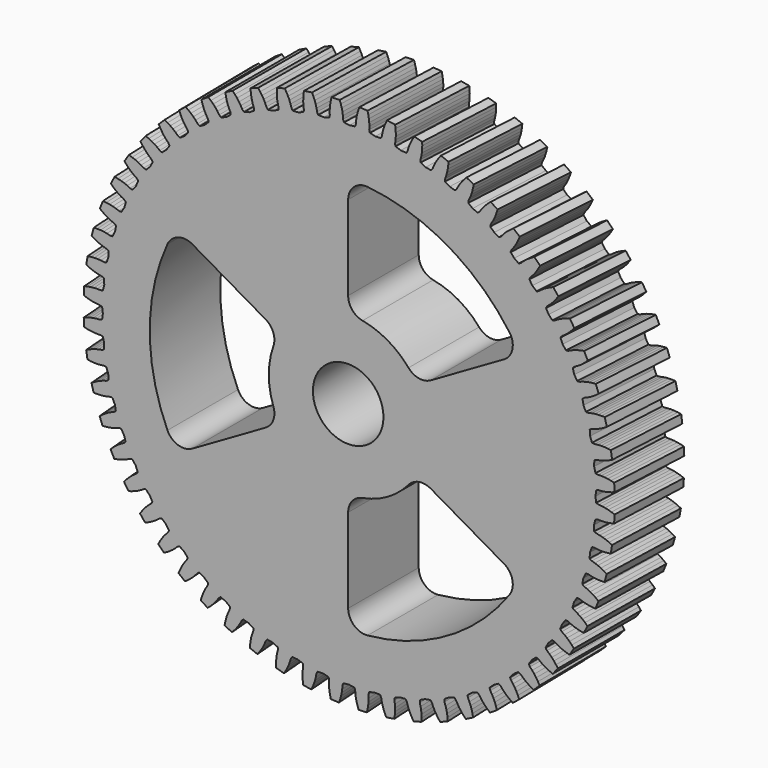
from build123d import *

# Parameters (mm, degrees)
F4_R     = 4
F5_DEPTH = 25
F7_DEPTH = 25


with BuildPart() as f3:
    # F0 (on Front) → F3 section 0
    with BuildSketch(Plane.XZ):
        Polygon((27.99593, -1.14699), (27.92323, -0.5264), (28.01927, 0.091), (28.1103, 0.13907), (28.29245, 0.18964), (28.65722, 0.21039), (29.02178, 0.25349), (29.38595, 0.32911), (29.74963, 0.42693), (30.11269, 0.54333), (30.08147, 1.47455), (29.71143, 1.56637), (29.34201, 1.63962), (28.9736, 1.69069), (28.60697, 1.70927), (28.24164, 1.70554), (28.0565, 1.74381), (27.96246, 1.78567), (27.82529, 2.39525), (27.85626, 3.01931), (27.94177, 3.07663), (28.11764, 3.14597), (28.47824, 3.20473), (28.8363, 3.2857), (29.19057, 3.39897), (29.54203, 3.53428), (29.89093, 3.68799), (29.76255, 4.61084), (29.38494, 4.66348), (29.00989, 4.69772), (28.63816, 4.70999), (28.27159, 4.69015), (27.90865, 4.64826), (27.72053, 4.66696), (27.62262, 4.69876), (27.42248, 5.29067), (27.38806, 5.91455), (27.4671, 5.98049), (27.63477, 6.06783), (27.98725, 6.16396), (28.33488, 6.28191), (28.67537, 6.4316), (29.01076, 6.6029), (29.34169, 6.79224), (29.11754, 7.69661), (28.7365, 7.7095), (28.35992, 7.70434), (27.98895, 7.67769), (27.62646, 7.61964), (27.26989, 7.54004), (27.08084, 7.53897), (26.98015, 7.56037), (26.71924, 8.12811), (26.61979, 8.74498), (26.69151, 8.81882), (26.84912, 8.92321), (27.18962, 9.05566), (27.52302, 9.2093), (27.846, 9.39376), (28.16165, 9.59918), (28.47097, 9.82207), (28.15352, 10.69806), (27.77321, 10.67105), (27.39924, 10.62655), (27.03308, 10.56127), (26.67865, 10.46565), (26.33235, 10.34922), (26.14445, 10.32839), (26.04208, 10.33914), (25.72325, 10.87651), (25.55986, 11.4796), (25.62347, 11.56053), (25.76931, 11.68082), (26.0941, 11.84814), (26.40962, 12.03579), (26.71154, 12.253), (27.00399, 12.49028), (27.28832, 12.74429), (26.88104, 13.5823), (26.50564, 13.51568), (26.13837, 13.43234), (25.78104, 13.32914), (25.43855, 13.197), (25.10631, 13.045), (24.92162, 13.00465), (24.81868, 13.00464), (24.44543, 13.50574), (24.2199, 14.08844), (24.2747, 14.17558), (24.40716, 14.31046), (24.71268, 14.51081), (25.00686, 14.73042), (25.28442, 14.97799), (25.55047, 15.24455), (25.80669, 15.52689), (25.31404, 16.31773), (24.94767, 16.21223), (24.59112, 16.09096), (24.24653, 15.95098), (23.91973, 15.78376), (23.6052, 15.59786), (23.42574, 15.53843), (23.32336, 15.52766), (22.89978, 15.98699), (22.61457, 16.54293), (22.65997, 16.63532), (22.77761, 16.78331), (23.06051, 17.0145), (23.33012, 17.26365), (23.58029, 17.53888), (23.81701, 17.83179), (24.04231, 18.13936), (23.4697, 18.87438), (23.11636, 18.73116), (22.77444, 18.57329), (22.44638, 18.39805), (22.13884, 18.19758), (21.84547, 17.97983), (21.6732, 17.90197), (21.57251, 17.88055), (21.10323, 18.29309), (20.76148, 18.81618), (20.79697, 18.9128), (20.8985, 19.07228), (21.15568, 19.33177), (21.39777, 19.60774), (21.6178, 19.90761), (21.82261, 20.22366), (22.01453, 20.5531), (21.36823, 21.22423), (21.03179, 21.04487), (20.70824, 20.85212), (20.40029, 20.64355), (20.1154, 20.41203), (19.84639, 20.16481), (19.68321, 20.06936), (19.58531, 20.03754), (19.07548, 20.39877), (18.68092, 20.88326), (18.70611, 20.98307), (18.79042, 21.15228), (19.01907, 21.43724), (19.23099, 21.737), (19.41846, 22.05823), (19.58911, 22.39395), (19.74555, 22.74165), (19.03263, 23.34155), (18.71678, 23.128), (18.41516, 22.90249), (18.1307, 22.66287), (17.87156, 22.40285), (17.62988, 22.12886), (17.47756, 22.01688), (17.38353, 21.975), (16.83873, 22.28095), (16.39569, 22.72155), (16.41031, 22.82345), (16.47647, 23.00054), (16.67408, 23.30784), (16.8535, 23.62811), (17.00637, 23.96717), (17.141, 24.3189), (17.26023, 24.68104), (16.48851, 25.20314), (16.19672, 24.95774), (15.92032, 24.70193), (15.66246, 24.4339), (15.43193, 24.14821), (15.2202, 23.85046), (15.08043, 23.72317), (14.99128, 23.67169), (14.41749, 23.91902), (13.93082, 24.3109), (13.93471, 24.41376), (13.98199, 24.5968), (14.14641, 24.92307), (14.29137, 25.26034), (14.40796, 25.61353), (14.50508, 25.9774), (14.5858, 26.35002), (13.76374, 26.78859), (13.4992, 26.51404), (13.25105, 26.23074), (13.02263, 25.93722), (12.82321, 25.629), (12.64377, 25.31075), (12.51807, 25.16955), (12.4348, 25.10903), (11.83829, 25.29503), (11.31333, 25.63389), (11.30644, 25.7366), (11.33433, 25.92358), (11.46374, 26.26524), (11.57265, 26.61582), (11.65169, 26.97926), (11.71024, 27.35128), (11.75157, 27.7303), (10.88817, 28.08054), (10.65377, 27.77984), (10.4366, 27.47216), (10.24011, 27.15637), (10.07401, 26.82899), (9.92882, 26.49373), (9.81856, 26.34016), (9.74207, 26.27127), (9.12939, 26.3939), (8.57188, 26.67603), (8.5543, 26.77745), (8.56249, 26.96632), (8.65547, 27.31965), (8.72714, 27.67969), (8.76776, 28.0494), (8.7871, 28.42551), (8.78859, 28.80677), (7.89331, 29.06484), (7.69163, 28.74128), (7.50781, 28.41259), (7.3454, 28.07798), (7.21443, 27.73504), (7.10508, 27.38643), (7.01148, 27.22218), (6.9426, 27.14568), (6.32047, 27.20359), (5.73652, 27.4259), (5.70843, 27.52493), (5.69684, 27.71362), (5.75238, 28.07473), (5.78602, 28.44029), (5.78777, 28.81222), (5.76769, 29.18829), (5.72932, 29.56762), (4.81196, 29.73069), (4.64521, 29.38783), (4.49675, 29.04172), (4.37021, 28.69197), (4.2758, 28.33722), (4.20349, 27.97909), (4.12757, 27.80596), (4.06708, 27.72267), (3.44229, 27.71524), (2.83831, 27.87529), (2.80002, 27.97084), (2.76877, 28.15729), (2.78626, 28.52222), (2.7815, 28.88929), (2.74436, 29.25937), (2.68509, 29.63128), (2.60728, 30.00452), (1.6779, 30.07081), (1.5479, 29.7124), (1.43643, 29.35266), (1.34714, 28.99161), (1.29034, 28.62893), (1.25585, 28.2652), (1.19845, 28.08508), (1.14699, 27.99593), (0.5264, 27.92323), (-0.091, 28.01927), (-0.13907, 28.1103), (-0.18964, 28.29245), (-0.21039, 28.65722), (-0.25349, 29.02178), (-0.32911, 29.38595), (-0.42693, 29.74963), (-0.54333, 30.11269), (-1.47455, 30.08147), (-1.56637, 29.71143), (-1.63962, 29.34201), (-1.69069, 28.9736), (-1.70927, 28.60697), (-1.70555, 28.24164), (-1.74381, 28.0565), (-1.78567, 27.96246), (-2.39525, 27.82529), (-3.01931, 27.85626), (-3.07663, 27.94177), (-3.14597, 28.11764), (-3.20473, 28.47824), (-3.2857, 28.8363), (-3.39897, 29.19057), (-3.53428, 29.54203), (-3.68799, 29.89093), (-4.61084, 29.76255), (-4.66348, 29.38494), (-4.69772, 29.00989), (-4.70999, 28.63816), (-4.69015, 28.27159), (-4.64826, 27.90865), (-4.66696, 27.72053), (-4.69876, 27.62262), (-5.29067, 27.42248), (-5.91455, 27.38806), (-5.98049, 27.4671), (-6.06783, 27.63477), (-6.16396, 27.98725), (-6.28192, 28.33488), (-6.4316, 28.67537), (-6.6029, 29.01076), (-6.79224, 29.34169), (-7.69661, 29.11754), (-7.7095, 28.7365), (-7.70434, 28.35992), (-7.67769, 27.98895), (-7.61964, 27.62646), (-7.54004, 27.26989), (-7.53898, 27.08084), (-7.56037, 26.98015), (-8.12811, 26.71924), (-8.74498, 26.61979), (-8.81882, 26.69151), (-8.92321, 26.84912), (-9.05566, 27.18962), (-9.2093, 27.52302), (-9.39376, 27.846), (-9.59918, 28.16165), (-9.82207, 28.47097), (-10.69806, 28.15352), (-10.67105, 27.77321), (-10.62656, 27.39924), (-10.56127, 27.03308), (-10.46565, 26.67865), (-10.34922, 26.33235), (-10.32839, 26.14445), (-10.33915, 26.04208), (-10.87651, 25.72325), (-11.4796, 25.55986), (-11.56053, 25.62347), (-11.68082, 25.76931), (-11.84814, 26.0941), (-12.03579, 26.40962), (-12.253, 26.71154), (-12.49029, 27.00399), (-12.74429, 27.28832), (-13.5823, 26.88104), (-13.51568, 26.50564), (-13.43234, 26.13837), (-13.32914, 25.78104), (-13.197, 25.43855), (-13.045, 25.10631), (-13.00465, 24.92162), (-13.00464, 24.81868), (-13.50574, 24.44543), (-14.08844, 24.2199), (-14.17558, 24.2747), (-14.31046, 24.40716), (-14.51081, 24.71268), (-14.73042, 25.00686), (-14.97799, 25.28442), (-15.24455, 25.55047), (-15.52689, 25.80669), (-16.31773, 25.31404), (-16.21223, 24.94767), (-16.09096, 24.59112), (-15.95098, 24.24653), (-15.78376, 23.91973), (-15.59786, 23.6052), (-15.53843, 23.42574), (-15.52766, 23.32336), (-15.98699, 22.89978), (-16.54293, 22.61457), (-16.63532, 22.65997), (-16.78331, 22.77761), (-17.0145, 23.06051), (-17.26365, 23.33012), (-17.53888, 23.58029), (-17.83179, 23.81701), (-18.13936, 24.04231), (-18.87438, 23.4697), (-18.73116, 23.11636), (-18.57329, 22.77444), (-18.39805, 22.44638), (-18.19758, 22.13884), (-17.97983, 21.84547), (-17.90197, 21.6732), (-17.88056, 21.57251), (-18.29309, 21.10323), (-18.81618, 20.76148), (-18.91281, 20.79697), (-19.07228, 20.8985), (-19.33177, 21.15568), (-19.60774, 21.39777), (-19.90761, 21.6178), (-20.22366, 21.82261), (-20.5531, 22.01453), (-21.22424, 21.36823), (-21.04487, 21.03179), (-20.85212, 20.70824), (-20.64355, 20.40029), (-20.41204, 20.1154), (-20.16481, 19.84639), (-20.06936, 19.68321), (-20.03755, 19.58531), (-20.39877, 19.07548), (-20.88327, 18.68092), (-20.98307, 18.70611), (-21.15229, 18.79042), (-21.43724, 19.01907), (-21.737, 19.23099), (-22.05823, 19.41846), (-22.39395, 19.58911), (-22.74165, 19.74555), (-23.34155, 19.03263), (-23.128, 18.71678), (-22.90249, 18.41516), (-22.66287, 18.1307), (-22.40285, 17.87156), (-22.12886, 17.62988), (-22.01688, 17.47756), (-21.975, 17.38353), (-22.28095, 16.83873), (-22.72155, 16.39569), (-22.82345, 16.41031), (-23.00054, 16.47647), (-23.30784, 16.67408), (-23.62811, 16.8535), (-23.96717, 17.00637), (-24.3189, 17.141), (-24.68104, 17.26023), (-25.20314, 16.48851), (-24.95774, 16.19672), (-24.70193, 15.92032), (-24.4339, 15.66246), (-24.14821, 15.43193), (-23.85046, 15.2202), (-23.72317, 15.08043), (-23.67169, 14.99128), (-23.91902, 14.41749), (-24.3109, 13.93082), (-24.41376, 13.93471), (-24.5968, 13.98199), (-24.92307, 14.14641), (-25.26034, 14.29137), (-25.61353, 14.40796), (-25.9774, 14.50508), (-26.35002, 14.5858), (-26.78859, 13.76374), (-26.51404, 13.4992), (-26.23074, 13.25105), (-25.93722, 13.02263), (-25.629, 12.82321), (-25.31075, 12.64377), (-25.16955, 12.51807), (-25.10903, 12.4348), (-25.29503, 11.83829), (-25.63389, 11.31333), (-25.7366, 11.30644), (-25.92358, 11.33433), (-26.26524, 11.46374), (-26.61582, 11.57265), (-26.97926, 11.65169), (-27.35129, 11.71024), (-27.7303, 11.75157), (-28.08054, 10.88817), (-27.77984, 10.65377), (-27.47216, 10.4366), (-27.15637, 10.24011), (-26.82899, 10.07401), (-26.49373, 9.92882), (-26.34016, 9.81856), (-26.27127, 9.74207), (-26.3939, 9.12939), (-26.67603, 8.57188), (-26.77745, 8.5543), (-26.96633, 8.56249), (-27.31965, 8.65547), (-27.67969, 8.72714), (-28.0494, 8.76776), (-28.42551, 8.7871), (-28.80677, 8.78859), (-29.06484, 7.89331), (-28.74128, 7.69163), (-28.41259, 7.50781), (-28.07799, 7.3454), (-27.73504, 7.21443), (-27.38644, 7.10508), (-27.22218, 7.01148), (-27.14568, 6.9426), (-27.20359, 6.32047), (-27.4259, 5.73652), (-27.52493, 5.70843), (-27.71362, 5.69684), (-28.07473, 5.75238), (-28.44029, 5.78602), (-28.81222, 5.78777), (-29.18829, 5.76769), (-29.56762, 5.72932), (-29.73069, 4.81196), (-29.38783, 4.64521), (-29.04172, 4.49675), (-28.69197, 4.37021), (-28.33722, 4.2758), (-27.97909, 4.20349), (-27.80596, 4.12757), (-27.72267, 4.06708), (-27.71524, 3.44229), (-27.87529, 2.83831), (-27.97084, 2.80002), (-28.15729, 2.76877), (-28.52222, 2.78626), (-28.8893, 2.7815), (-29.25937, 2.74436), (-29.63128, 2.68509), (-30.00452, 2.60728), (-30.07081, 1.6779), (-29.7124, 1.5479), (-29.35266, 1.43643), (-28.99161, 1.34714), (-28.62893, 1.29034), (-28.2652, 1.25585), (-28.08508, 1.19845), (-27.99593, 1.14699), (-27.92323, 0.5264), (-28.01927, -0.091), (-28.1103, -0.13907), (-28.29245, -0.18964), (-28.65722, -0.21039), (-29.02178, -0.25349), (-29.38595, -0.32911), (-29.74963, -0.42693), (-30.11269, -0.54333), (-30.08147, -1.47455), (-29.71143, -1.56637), (-29.34201, -1.63962), (-28.9736, -1.69069), (-28.60697, -1.70927), (-28.24164, -1.70555), (-28.0565, -1.74381), (-27.96246, -1.78567), (-27.82529, -2.39525), (-27.85626, -3.01931), (-27.94177, -3.07663), (-28.11764, -3.14597), (-28.47824, -3.20473), (-28.8363, -3.2857), (-29.19057, -3.39897), (-29.54203, -3.53428), (-29.89093, -3.68799), (-29.76255, -4.61084), (-29.38494, -4.66348), (-29.00989, -4.69772), (-28.63816, -4.70999), (-28.27159, -4.69015), (-27.90865, -4.64826), (-27.72053, -4.66696), (-27.62262, -4.69876), (-27.42248, -5.29067), (-27.38806, -5.91455), (-27.46711, -5.98049), (-27.63477, -6.06783), (-27.98725, -6.16396), (-28.33488, -6.28192), (-28.67537, -6.4316), (-29.01076, -6.6029), (-29.34169, -6.79224), (-29.11754, -7.69661), (-28.7365, -7.7095), (-28.35992, -7.70434), (-27.98895, -7.67769), (-27.62646, -7.61964), (-27.26989, -7.54004), (-27.08084, -7.53898), (-26.98015, -7.56037), (-26.71924, -8.12811), (-26.61979, -8.74498), (-26.69151, -8.81882), (-26.84912, -8.92321), (-27.18962, -9.05566), (-27.52302, -9.2093), (-27.846, -9.39376), (-28.16165, -9.59918), (-28.47097, -9.82207), (-28.15352, -10.69806), (-27.77321, -10.67105), (-27.39924, -10.62656), (-27.03308, -10.56127), (-26.67865, -10.46565), (-26.33235, -10.34922), (-26.14445, -10.32839), (-26.04208, -10.33915), (-25.72325, -10.87651), (-25.55986, -11.4796), (-25.62347, -11.56053), (-25.76931, -11.68082), (-26.0941, -11.84814), (-26.40962, -12.03579), (-26.71154, -12.253), (-27.00399, -12.49029), (-27.28832, -12.74429), (-26.88104, -13.5823), (-26.50564, -13.51568), (-26.13837, -13.43234), (-25.78104, -13.32914), (-25.43855, -13.197), (-25.10631, -13.045), (-24.92162, -13.00465), (-24.81868, -13.00464), (-24.44543, -13.50574), (-24.2199, -14.08844), (-24.2747, -14.17558), (-24.40716, -14.31046), (-24.71268, -14.51081), (-25.00686, -14.73042), (-25.28442, -14.97799), (-25.55047, -15.24455), (-25.80669, -15.52689), (-25.31405, -16.31773), (-24.94767, -16.21223), (-24.59112, -16.09096), (-24.24653, -15.95098), (-23.91973, -15.78376), (-23.6052, -15.59786), (-23.42574, -15.53843), (-23.32336, -15.52766), (-22.89978, -15.98699), (-22.61457, -16.54293), (-22.65997, -16.63532), (-22.77761, -16.78331), (-23.06051, -17.0145), (-23.33012, -17.26365), (-23.58029, -17.53888), (-23.81701, -17.83179), (-24.04231, -18.13936), (-23.4697, -18.87438), (-23.11636, -18.73116), (-22.77444, -18.57329), (-22.44638, -18.39805), (-22.13884, -18.19758), (-21.84547, -17.97983), (-21.6732, -17.90197), (-21.57251, -17.88056), (-21.10324, -18.29309), (-20.76148, -18.81618), (-20.79697, -18.91281), (-20.8985, -19.07228), (-21.15568, -19.33177), (-21.39777, -19.60774), (-21.6178, -19.90761), (-21.82261, -20.22366), (-22.01453, -20.5531), (-21.36823, -21.22424), (-21.03179, -21.04487), (-20.70824, -20.85212), (-20.40029, -20.64355), (-20.1154, -20.41204), (-19.84639, -20.16481), (-19.68321, -20.06936), (-19.58531, -20.03755), (-19.07548, -20.39877), (-18.68092, -20.88327), (-18.70611, -20.98307), (-18.79042, -21.15229), (-19.01907, -21.43724), (-19.23099, -21.737), (-19.41846, -22.05823), (-19.58911, -22.39395), (-19.74555, -22.74165), (-19.03263, -23.34155), (-18.71678, -23.128), (-18.41516, -22.90249), (-18.1307, -22.66287), (-17.87156, -22.40285), (-17.62988, -22.12886), (-17.47756, -22.01688), (-17.38353, -21.975), (-16.83873, -22.28095), (-16.39569, -22.72155), (-16.41031, -22.82345), (-16.47647, -23.00054), (-16.67408, -23.30784), (-16.8535, -23.62811), (-17.00637, -23.96717), (-17.141, -24.3189), (-17.26023, -24.68104), (-16.48851, -25.20314), (-16.19672, -24.95774), (-15.92032, -24.70193), (-15.66246, -24.4339), (-15.43193, -24.14821), (-15.2202, -23.85046), (-15.08043, -23.72317), (-14.99128, -23.67169), (-14.41749, -23.91902), (-13.93082, -24.3109), (-13.93471, -24.41376), (-13.98199, -24.5968), (-14.14641, -24.92307), (-14.29137, -25.26034), (-14.40796, -25.61353), (-14.50508, -25.9774), (-14.5858, -26.35002), (-13.76374, -26.78859), (-13.4992, -26.51404), (-13.25105, -26.23074), (-13.02263, -25.93722), (-12.82321, -25.629), (-12.64377, -25.31075), (-12.51807, -25.16955), (-12.4348, -25.10903), (-11.83829, -25.29503), (-11.31333, -25.63389), (-11.30645, -25.7366), (-11.33433, -25.92358), (-11.46374, -26.26524), (-11.57265, -26.61582), (-11.65169, -26.97926), (-11.71024, -27.35129), (-11.75157, -27.7303), (-10.88817, -28.08054), (-10.65377, -27.77984), (-10.4366, -27.47216), (-10.24011, -27.15637), (-10.07401, -26.82899), (-9.92882, -26.49373), (-9.81856, -26.34016), (-9.74207, -26.27127), (-9.12939, -26.3939), (-8.57188, -26.67603), (-8.5543, -26.77745), (-8.56249, -26.96633), (-8.65547, -27.31965), (-8.72714, -27.67969), (-8.76776, -28.0494), (-8.7871, -28.42551), (-8.78859, -28.80677), (-7.89331, -29.06484), (-7.69163, -28.74128), (-7.50781, -28.41259), (-7.3454, -28.07799), (-7.21443, -27.73504), (-7.10508, -27.38644), (-7.01148, -27.22218), (-6.9426, -27.14568), (-6.32047, -27.20359), (-5.73652, -27.4259), (-5.70843, -27.52493), (-5.69684, -27.71362), (-5.75238, -28.07473), (-5.78602, -28.44029), (-5.78777, -28.81222), (-5.76769, -29.18829), (-5.72932, -29.56762), (-4.81197, -29.73069), (-4.64521, -29.38783), (-4.49675, -29.04172), (-4.37021, -28.69197), (-4.27581, -28.33722), (-4.20349, -27.97909), (-4.12757, -27.80596), (-4.06708, -27.72267), (-3.44229, -27.71524), (-2.83831, -27.87529), (-2.80002, -27.97084), (-2.76877, -28.15729), (-2.78626, -28.52222), (-2.7815, -28.8893), (-2.74436, -29.25937), (-2.68509, -29.63128), (-2.60728, -30.00452), (-1.6779, -30.07081), (-1.5479, -29.7124), (-1.43644, -29.35266), (-1.34714, -28.99161), (-1.29034, -28.62893), (-1.25585, -28.2652), (-1.19845, -28.08508), (-1.14699, -27.99593), (-0.5264, -27.92323), (0.091, -28.01927), (0.13907, -28.1103), (0.18964, -28.29245), (0.21039, -28.65722), (0.25349, -29.02178), (0.32911, -29.38595), (0.42693, -29.74963), (0.54333, -30.11269), (1.47455, -30.08147), (1.56637, -29.71143), (1.63962, -29.34201), (1.69069, -28.9736), (1.70927, -28.60697), (1.70554, -28.24164), (1.74381, -28.0565), (1.78567, -27.96246), (2.39525, -27.82529), (3.01931, -27.85626), (3.07663, -27.94177), (3.14597, -28.11764), (3.20473, -28.47824), (3.2857, -28.8363), (3.39897, -29.19057), (3.53428, -29.54203), (3.68799, -29.89093), (4.61084, -29.76255), (4.66348, -29.38494), (4.69772, -29.00989), (4.70999, -28.63816), (4.69015, -28.27159), (4.64826, -27.90865), (4.66696, -27.72053), (4.69876, -27.62262), (5.29067, -27.42248), (5.91455, -27.38806), (5.98049, -27.46711), (6.06783, -27.63477), (6.16396, -27.98725), (6.28191, -28.33488), (6.4316, -28.67537), (6.6029, -29.01076), (6.79224, -29.34169), (7.69661, -29.11754), (7.7095, -28.7365), (7.70434, -28.35992), (7.67769, -27.98895), (7.61964, -27.62646), (7.54004, -27.26989), (7.53897, -27.08084), (7.56037, -26.98015), (8.12811, -26.71924), (8.74498, -26.61979), (8.81882, -26.69151), (8.92321, -26.84912), (9.05566, -27.18962), (9.2093, -27.52302), (9.39376, -27.846), (9.59918, -28.16165), (9.82207, -28.47097), (10.69806, -28.15352), (10.67105, -27.77321), (10.62655, -27.39924), (10.56127, -27.03308), (10.46565, -26.67865), (10.34922, -26.33235), (10.32839, -26.14445), (10.33914, -26.04208), (10.87651, -25.72325), (11.4796, -25.55986), (11.56053, -25.62347), (11.68082, -25.76931), (11.84814, -26.0941), (12.03579, -26.40962), (12.253, -26.71154), (12.49028, -27.00399), (12.74429, -27.28832), (13.5823, -26.88104), (13.51568, -26.50564), (13.43234, -26.13837), (13.32914, -25.78104), (13.197, -25.43855), (13.045, -25.10631), (13.00465, -24.92162), (13.00464, -24.81868), (13.50574, -24.44543), (14.08844, -24.2199), (14.17558, -24.2747), (14.31046, -24.40716), (14.51081, -24.71268), (14.73042, -25.00686), (14.97799, -25.28442), (15.24455, -25.55047), (15.52689, -25.80669), (16.31773, -25.31405), (16.21223, -24.94767), (16.09096, -24.59112), (15.95098, -24.24653), (15.78376, -23.91973), (15.59786, -23.6052), (15.53843, -23.42574), (15.52766, -23.32336), (15.98699, -22.89978), (16.54293, -22.61457), (16.63532, -22.65997), (16.78331, -22.77761), (17.0145, -23.06051), (17.26365, -23.33012), (17.53888, -23.58029), (17.83179, -23.81701), (18.13936, -24.04231), (18.87438, -23.4697), (18.73116, -23.11636), (18.57329, -22.77444), (18.39805, -22.44638), (18.19758, -22.13884), (17.97983, -21.84547), (17.90197, -21.6732), (17.88055, -21.57251), (18.29309, -21.10324), (18.81618, -20.76148), (18.9128, -20.79697), (19.07228, -20.8985), (19.33177, -21.15568), (19.60774, -21.39777), (19.90761, -21.6178), (20.22366, -21.82261), (20.5531, -22.01453), (21.22423, -21.36823), (21.04487, -21.03179), (20.85212, -20.70824), (20.64355, -20.40029), (20.41203, -20.1154), (20.16481, -19.84639), (20.06936, -19.68321), (20.03754, -19.58531), (20.39877, -19.07548), (20.88326, -18.68092), (20.98307, -18.70611), (21.15228, -18.79042), (21.43724, -19.01907), (21.737, -19.23099), (22.05823, -19.41846), (22.39395, -19.58911), (22.74165, -19.74555), (23.34155, -19.03263), (23.128, -18.71678), (22.90249, -18.41516), (22.66287, -18.1307), (22.40285, -17.87156), (22.12886, -17.62988), (22.01688, -17.47756), (21.975, -17.38353), (22.28095, -16.83873), (22.72155, -16.39569), (22.82345, -16.41031), (23.00054, -16.47647), (23.30784, -16.67408), (23.62811, -16.8535), (23.96717, -17.00637), (24.3189, -17.141), (24.68104, -17.26023), (25.20314, -16.48851), (24.95774, -16.19672), (24.70193, -15.92032), (24.4339, -15.66246), (24.14821, -15.43193), (23.85046, -15.2202), (23.72317, -15.08043), (23.67169, -14.99128), (23.91902, -14.41749), (24.3109, -13.93082), (24.41376, -13.93471), (24.5968, -13.98199), (24.92307, -14.14641), (25.26034, -14.29137), (25.61353, -14.40796), (25.9774, -14.50508), (26.35002, -14.5858), (26.78859, -13.76374), (26.51404, -13.4992), (26.23074, -13.25105), (25.93722, -13.02263), (25.629, -12.82321), (25.31075, -12.64377), (25.16955, -12.51807), (25.10903, -12.4348), (25.29503, -11.83829), (25.63389, -11.31333), (25.7366, -11.30645), (25.92358, -11.33433), (26.26524, -11.46374), (26.61582, -11.57265), (26.97926, -11.65169), (27.35128, -11.71024), (27.7303, -11.75157), (28.08054, -10.88817), (27.77984, -10.65377), (27.47216, -10.4366), (27.15637, -10.24011), (26.82899, -10.07401), (26.49373, -9.92882), (26.34016, -9.81856), (26.27127, -9.74207), (26.3939, -9.12939), (26.67603, -8.57188), (26.77745, -8.5543), (26.96632, -8.56249), (27.31965, -8.65547), (27.67969, -8.72714), (28.0494, -8.76776), (28.42551, -8.7871), (28.80677, -8.78859), (29.06484, -7.89331), (28.74128, -7.69163), (28.41259, -7.50781), (28.07798, -7.3454), (27.73504, -7.21443), (27.38643, -7.10508), (27.22218, -7.01148), (27.14568, -6.9426), (27.20359, -6.32047), (27.4259, -5.73652), (27.52493, -5.70843), (27.71362, -5.69684), (28.07473, -5.75238), (28.44029, -5.78602), (28.81222, -5.78777), (29.18829, -5.76769), (29.56762, -5.72932), (29.73069, -4.81197), (29.38783, -4.64521), (29.04172, -4.49675), (28.69197, -4.37021), (28.33722, -4.27581), (27.97909, -4.20349), (27.80596, -4.12757), (27.72267, -4.06708), (27.71524, -3.44229), (27.87529, -2.83831), (27.97084, -2.80002), (28.15729, -2.76877), (28.52222, -2.78626), (28.88929, -2.7815), (29.25937, -2.74436), (29.63128, -2.68509), (30.00452, -2.60728), (30.07081, -1.6779), (29.7124, -1.5479), (29.35266, -1.43644), (28.99161, -1.34714), (28.62893, -1.29034), (28.2652, -1.25585), (28.08508, -1.19845), align=None)
    # F2 (on offset) → F3 section 1
    with BuildSketch(Plane.XZ.offset(10)):
        Polygon((27.902526891, -3.6338677754), (27.8841915189, -3.0093030852), (28.0336760132, -2.4026229161), (28.1285491932, -2.3626696243), (28.3144135233, -2.3281674769), (28.679603945, -2.3392882372), (29.0465330967, -2.3281257433), (29.4159080371, -2.2845330071), (29.7867296997, -2.2187820422), (30.1585530752, -2.1344677433), (30.2086130475, -1.2040703143), (29.8479838017, -1.0803486061), (29.4863537145, -0.9751802699), (29.1237966696, -0.8921955595), (28.7601811611, -0.8417323521), (28.3959162611, -0.8136075508), (28.214816225, -0.7593471655), (28.124782415, -0.7094503294), (28.0412627859, -0.0902348121), (28.1265053485, 0.5287512379), (28.2166857244, 0.5784004304), (28.3979298651, 0.6321484903), (28.7622789447, 0.6592565299), (29.1260334188, 0.7087114294), (29.4888274454, 0.7906737378), (29.8507430776, 0.8948370851), (30.211712117, 1.0175535335), (30.1642523188, 1.9480808649), (29.7926671172, 2.0334314338), (29.4220285083, 2.1002289016), (29.0527824541, 2.1448506148), (28.6858781937, 2.1570347926), (28.3206683359, 2.146936502), (28.1348940017, 2.1819610811), (28.0401281314, 2.2221734913), (27.8923380803, 2.8292744454), (27.9124237835, 3.4537802943), (27.9969100621, 3.5125805828), (28.1715542097, 3.5849748243), (28.5310711985, 3.6500183645), (28.8876583812, 3.7372215783), (29.2398990571, 3.8566663038), (29.5889425756, 3.998083291), (29.9351153554, 4.1578603452), (29.7906393529, 5.078324904), (29.4121727627, 5.1243756779), (29.0365760396, 5.1520564229), (28.6646949919, 5.15784), (28.298524985, 5.131603983), (27.9363742443, 5.0833840082), (27.74795038, 5.0987948731), (27.6495086688, 5.1288891514), (27.4390733115, 5.7172085341), (27.3937655118, 6.3403987961), (27.4716481756, 6.4077070028), (27.6377566099, 6.4979631507), (27.9885046827, 6.600232608), (28.3340266034, 6.7242302368), (28.6718543153, 6.879838749), (29.0042067044, 7.0569663537), (29.3317757919, 7.2520491756), (29.0918813441, 8.1523733597), (28.7106644619, 8.1586123415), (28.3342391001, 8.1468753105), (27.9637829225, 8.1137566674), (27.6023678036, 8.0493911403), (27.2472380365, 7.9635862253), (27.0582375986, 7.9592120538), (26.9571940716, 7.9788432802), (26.6864121975, 8.5419562905), (26.5762067027, 9.1569917278), (26.6466281617, 9.2320697879), (26.8023971607, 9.3391912547), (27.1405341356, 9.4775672379), (27.4712082619, 9.637003793), (27.790910464, 9.8270731815), (28.1029279181, 10.0379615625), (28.4083143868, 10.2662239854), (28.0756215942, 11.1365418953), (27.6958437889, 11.1028936703), (27.3227078025, 11.0518804938), (26.9577430784, 10.9802165625), (26.6050395964, 10.8784293655), (26.260816197, 10.7559643953), (26.073312264, 10.7318647334), (25.9707631102, 10.7408265836), (25.6426071819, 11.2725506278), (25.4687210429, 11.872689513), (25.5309072638, 11.9547217843), (25.6746187801, 12.0775438755), (25.9964378373, 12.2505036608), (26.3086386663, 12.443638502), (26.6067196139, 12.6660754755), (26.8949894481, 12.9084333488), (27.1748420061, 13.1673679155), (26.7529929356, 13.9981358072), (26.3788221532, 13.924968516), (26.0130595567, 13.835235365), (25.6575807648, 13.7258210286), (25.3174501542, 13.5877198479), (24.9879147832, 13.4299403493), (24.8039580169, 13.386377468), (24.7010289364, 13.384571456), (24.3190940335, 13.8790709962), (24.0834227072, 14.4577531661), (24.1367022656, 14.5458347235), (24.2667927883, 14.6830085753), (24.5687658045, 14.8886624679), (24.8590647104, 15.1133663172), (25.1322706131, 15.3657452317), (25.3936186106, 15.6369091133), (25.6448677679, 15.9236725278), (25.1384979359, 16.7058018046), (24.7740200558, 16.5939224101), (24.4196418875, 16.4664534447), (24.0775570825, 16.3204725988), (23.7537152533, 16.1475693248), (23.4424834517, 15.9562168095), (23.2640830449, 15.8936674101), (23.1619093248, 15.8811046314), (22.730370307, 16.3329752391), (22.4355110664, 16.8838601988), (22.4792870041, 16.9770193733), (22.5943302496, 17.1270435811), (22.8731476457, 17.3631314294), (23.1383687905, 17.6169517465), (23.3836969025, 17.8965037725), (23.6152731111, 18.1935007392), (23.8351753855, 18.5049601904), (23.2498275857, 19.2298650947), (22.8990355875, 19.0805102917), (22.5599175235, 18.9166930042), (22.234961293, 18.735756287), (21.9309770879, 18.5299470901), (21.6414441094, 18.3071136032), (21.4705660429, 18.2262488933), (21.3702652863, 18.2030825252), (20.8938586123, 18.6073725484), (20.543026118, 19.1244070875), (20.5768192771, 19.2216418272), (20.6755560754, 19.3828598313), (20.9281718935, 19.6468073119), (21.1654112794, 19.9269565896), (21.3801649387, 20.2306251254), (21.5794254899, 20.5501944819), (21.7655742402, 20.8829367341), (21.1076518461, 21.5426890056), (20.7743916419, 21.3574797692), (20.4542649055, 21.1591158179), (20.1500031026, 20.9451999669), (19.8691869723, 20.7087549607), (19.6045468357, 20.4568713753), (19.4430467592, 20.3585930557), (19.3457244892, 20.3250676763), (18.8296629172, 20.6773358928), (18.4267096384, 21.154872757), (18.4501551751, 21.2551107798), (18.5314978268, 21.425760675), (18.7551388208, 21.7146684594), (18.9617894433, 22.018082252), (19.1436287529, 22.3425285279), (19.3084017345, 22.6811863114), (19.4587406091, 23.0315566802), (18.73546125, 23.6189297618), (18.4233935797, 23.3998947571), (18.1257500546, 23.1691480387), (17.845510936, 22.9246119536), (17.5909586481, 22.6601011037), (17.3540837223, 22.3819376177), (17.2037515349, 22.2673137528), (17.1104539999, 22.2237995842), (16.5604036739, 22.5201975125), (16.1097401927, 22.9530023761), (16.1225802298, 23.0551319269), (16.1856333022, 23.2333546809), (16.3778639387, 23.5440529778), (16.5516673395, 23.8674054672), (16.6985962161, 24.2090899846), (16.8270600053, 24.5631107836), (16.9399488142, 24.9272776405), (16.1592408948, 25.4358259991), (15.8717789402, 25.1853769249), (15.5998820039, 24.9247826645), (15.3467492574, 24.6522877115), (15.1212249676, 24.3626211799), (14.9147304759, 24.0612214437), (14.7772024115, 23.9315142292), (14.6889746134, 23.8784819847), (14.1109454822, 24.1157634707), (13.6175167085, 24.4990872848), (13.6196046933, 24.6020069453), (13.6636849442, 24.7858446563), (13.8223801312, 25.1149257122), (13.9614307561, 25.4546795175), (14.0718458681, 25.8098477287), (14.1625967471, 26.1753491115), (14.2368032436, 26.5493246791), (13.4072141686, 26.9734821785), (13.1474983995, 26.6943557389), (12.904338718, 26.4067741668), (12.6810735098, 26.109311075), (12.4870725234, 25.7976534236), (12.3132151809, 25.4763233314), (12.189990246, 25.3329475038), (12.1077871545, 25.2709861938), (11.5081264956, 25.4465481301), (10.9773272391, 25.7761947384), (10.9686534718, 25.8787610027), (10.9932734115, 26.0661984898), (11.1166943331, 26.4100802215), (11.2194711607, 26.7625037085), (11.292158939, 27.1272665841), (11.3442054909, 27.5002597799), (11.3789188195, 27.8799391084), (10.5095379127, 28.2150558675), (10.2804252538, 27.9103046812), (10.0686575234, 27.5988864145), (9.8777023594, 27.2797046708), (9.7173415493, 26.9494844486), (9.5780242956, 26.6117314954), (9.4704651411, 26.4562642938), (9.395179836, 26.3860586869), (8.7804644175, 26.4979705241), (8.2181121168, 26.7703291634), (8.1987600409, 26.8714305292), (8.2036595614, 27.0604126418), (8.2904610252, 27.4153078793), (8.3558336682, 27.776544894), (8.3899928443, 28.1469070655), (8.402765915, 28.5232960929), (8.3976027123, 28.9045267936), (7.497946031, 29.1469294552), (7.3019483472, 28.8199073611), (7.1238878082, 28.4880535557), (6.96734661, 28.1506631477), (6.8423773689, 27.8054914523), (6.7391294441, 27.4550264768), (6.6484090689, 27.2891721527), (6.5808900498, 27.2114711472), (5.9578299972, 27.2585234571), (5.3700976, 27.470604744), (5.3402810363, 27.5691283408), (5.3254001402, 27.7575924592), (5.3746293307, 28.1196094365), (5.4018797024, 28.4856974856), (5.3971356286, 28.8576061838), (5.3705052611, 29.2332666748), (5.3255213611, 29.6118679723), (4.4054554867, 29.758906523), (4.2447126862, 29.4131906278), (4.1023134563, 29.0645347978), (3.9818956508, 28.7126408383), (3.8937021472, 28.3562913914), (3.8276422338, 27.9969514954), (3.7547621657, 27.822519646), (3.6957280521, 27.7381939232), (3.0711633619, 27.719858551), (2.4644831928, 27.8693430454), (2.4245299009, 27.9642162253), (2.3900277536, 28.1500805555), (2.4011485139, 28.5152709772), (2.38998602, 28.8822001288), (2.3463932838, 29.2515750693), (2.2806423189, 29.6223967319), (2.19632802, 29.9942201074), (1.265930591, 30.0442800797), (1.1422088827, 29.6836508339), (1.0370405466, 29.3220207467), (0.9540558362, 28.9594637018), (0.9035926287, 28.5958481933), (0.8754578655, 28.2315841649), (0.8212074422, 28.0504832572), (0.7713106061, 27.9604494472), (0.1520950888, 27.8769298181), (-0.4668909612, 27.9621723807), (-0.5165401537, 28.0523527565), (-0.5702882136, 28.2335968973), (-0.5973962532, 28.5979459769), (-0.6468511527, 28.961700451), (-0.7288134611, 29.3244944776), (-0.8329768084, 29.6864101098), (-0.9556932568, 30.0473791492), (-1.8862205882, 29.999919351), (-1.9715711571, 29.6283341494), (-2.0383686249, 29.2576955405), (-2.0829903381, 28.8884494863), (-2.0951745159, 28.5215452259), (-2.0850762253, 28.1563353681), (-2.1201008045, 27.9705610339), (-2.1603132146, 27.8757951636), (-2.7674141687, 27.7280051124), (-3.3919200176, 27.7480908157), (-3.4507203061, 27.8325770943), (-3.5231145477, 28.0072212419), (-3.5881580878, 28.3667382307), (-3.6753712635, 28.723326285), (-3.7948060271, 29.0755660893), (-3.9362230143, 29.4246096078), (-4.0960000685, 29.7707823876), (-5.0164646273, 29.6263063851), (-5.0625154012, 29.2478397949), (-5.0901961462, 28.8722430718), (-5.0959797234, 28.5003620241), (-5.0697437063, 28.1341920171), (-5.0215237316, 27.7720412765), (-5.0369445583, 27.5836182838), (-5.0670288747, 27.485175701), (-5.6553482574, 27.2747403437), (-6.2785385194, 27.229432544), (-6.3458467261, 27.3073152078), (-6.436102874, 27.4734236421), (-6.5383723313, 27.8241717149), (-6.6623699601, 28.1696936356), (-6.8179784723, 28.5075213475), (-6.995106077, 28.8398737366), (-7.1901888989, 29.1674428241), (-8.0905130831, 28.9275483763), (-8.0967520648, 28.5463314941), (-8.0850249958, 28.1699070038), (-8.0518963907, 27.7994499547), (-7.9875308636, 27.4380348358), (-7.9017259486, 27.0829050687), (-7.8973517771, 26.8939046308), (-7.9169929654, 26.7928619753), (-8.4800960139, 26.5220792297), (-9.0951314511, 26.4118737348), (-9.1702095113, 26.4822951939), (-9.277330978, 26.6380641929), (-9.4157069612, 26.9762011678), (-9.5751435163, 27.3068752941), (-9.7652129048, 27.6265774962), (-9.9761112478, 27.9385958218), (-10.2043637088, 28.243981419), (-11.0746816186, 27.9112886263), (-11.0410333937, 27.5315108211), (-10.9900202172, 27.1583748347), (-10.9183562859, 26.7934101106), (-10.8165690888, 26.4407066286), (-10.6941041187, 26.0964832292), (-10.6700044567, 25.9089792962), (-10.6789663069, 25.8064301424), (-11.2106903511, 25.4782742141), (-11.8108292364, 25.3043880751), (-11.8928615077, 25.366574296), (-12.0156835988, 25.5102858123), (-12.1886433841, 25.8321048695), (-12.3817782253, 26.1443056984), (-12.6042151988, 26.4423866461), (-12.8465730721, 26.7306564803), (-13.1055076388, 27.0105090382), (-13.9362755305, 26.5886599678), (-13.8631082393, 26.2144891854), (-13.7733750884, 25.8487265889), (-13.6639607519, 25.493247797), (-13.5258595712, 25.1531171864), (-13.3680800726, 24.8235818154), (-13.3245171913, 24.6396250491), (-13.3227111794, 24.5366959686), (-13.8172107195, 24.1547610657), (-14.3958928894, 23.9190897394), (-14.4839744468, 23.9723692978), (-14.6211482986, 24.1024598204), (-14.8268021912, 24.4044328367), (-15.0515060405, 24.6947317426), (-15.3038849551, 24.9679376453), (-15.5750488367, 25.2292856428), (-15.8618122511, 25.4805348001), (-16.643941528, 24.974164968), (-16.5320621334, 24.6096870879), (-16.404593168, 24.2553089197), (-16.2586123221, 23.9132241146), (-16.0857090481, 23.5893822854), (-15.8943565328, 23.2781504839), (-15.8318071334, 23.0997500771), (-15.8192543167, 22.9975772285), (-16.2711149624, 22.5660373391), (-16.8219999222, 22.2711780985), (-16.9151690585, 22.3149549078), (-17.0651833045, 22.4299972818), (-17.3012711528, 22.7088146779), (-17.5550914698, 22.9740358227), (-17.8346434959, 23.2193639347), (-18.1316404625, 23.4509401433), (-18.4430999137, 23.6708424177), (-19.1680147799, 23.0854954895), (-19.018650015, 22.7347026197), (-18.8548327275, 22.3955845557), (-18.6738960103, 22.0706283252), (-18.4680967753, 21.7666449916), (-18.2452533265, 21.4771111416), (-18.1643886166, 21.3062330751), (-18.1412322105, 21.20593319), (-18.5455122717, 20.7295256445), (-19.0625567728, 20.3786940218), (-19.1597815505, 20.4124863093), (-19.3210095166, 20.5112239791), (-19.5849470353, 20.7638389257), (-19.865096313, 21.0010783116), (-20.1687648487, 21.2158319709), (-20.4883342053, 21.4150925221), (-20.8210764574, 21.6012412724), (-21.4808287289, 20.9433188783), (-21.2956194925, 20.6100586741), (-21.0972555412, 20.2899319377), (-20.8833396903, 19.9856701348), (-20.646894684, 19.7048540045), (-20.3950110986, 19.4402138679), (-20.2967327791, 19.2787137914), (-20.2632073996, 19.1813915214), (-20.6154756161, 18.6653299494), (-21.0930124804, 18.2623766706), (-21.1932505031, 18.2858222073), (-21.3639003983, 18.367164859), (-21.6528081827, 18.590805853), (-21.9562219753, 18.7974564755), (-22.2806682512, 18.9792957851), (-22.6193260347, 19.1440687667), (-22.9696964035, 19.2944076413), (-23.5570694852, 18.5711282821), (-23.3380344804, 18.2590606119), (-23.107287762, 17.9614170868), (-22.8627516769, 17.6811779682), (-22.598240827, 17.4266256803), (-22.320077341, 17.1897507545), (-22.2054534761, 17.0394185671), (-22.1619393075, 16.9461210321), (-22.4583372358, 16.3960707061), (-22.8911420994, 15.9454072249), (-22.9932716502, 15.9582472619), (-23.1714944042, 16.0213003344), (-23.4821927012, 16.2135309709), (-23.8055451905, 16.3873343717), (-24.1472297079, 16.5342632483), (-24.5012505069, 16.6627270375), (-24.8654173638, 16.7756158464), (-25.3739657224, 15.994907927), (-25.1235166482, 15.7074459724), (-24.8629223878, 15.4355490361), (-24.5904274348, 15.1824162896), (-24.3007609032, 14.9568919998), (-23.999361167, 14.7503975081), (-23.8696539525, 14.6128694436), (-23.8166217081, 14.5246416456), (-24.053903194, 13.9466125144), (-24.4372270081, 13.4531837407), (-24.5401466686, 13.4552717255), (-24.7239843796, 13.4993519764), (-25.0530654355, 13.6580471634), (-25.3928192408, 13.7970977882), (-25.747987452, 13.9075129003), (-26.1134987968, 13.9982646509), (-26.4874644024, 14.0724702758), (-26.9116219018, 13.2428812008), (-26.6324954622, 12.9831654317), (-26.3449138901, 12.7400057502), (-26.0474507983, 12.516740542), (-25.7357931469, 12.3227395556), (-25.4144630547, 12.148882213), (-25.2710872271, 12.0256572782), (-25.2091259171, 11.9434541866), (-25.3846878534, 11.3437935278), (-25.7143344617, 10.8129942713), (-25.816900726, 10.804320504), (-26.004348175, 10.8289413152), (-26.3482199448, 10.9523613653), (-26.7006434318, 11.0551381929), (-27.0654063074, 11.1278259712), (-27.4383995032, 11.1798725231), (-27.8180788317, 11.2145858516), (-28.1531955909, 10.3452049449), (-27.8484444045, 10.116092286), (-27.5370261379, 9.9043245555), (-27.217854356, 9.7133702631), (-26.887624172, 9.5530085815), (-26.5498811807, 9.4136921994), (-26.3944040171, 9.3061321733), (-26.3241984102, 9.2308468682), (-26.4361102475, 8.6161314497), (-26.7084688868, 8.053779149), (-26.8095702525, 8.0344270731), (-26.9985523652, 8.0393265936), (-27.3534476026, 8.1261280574), (-27.7146846173, 8.1915007004), (-28.0850467888, 8.2256598765), (-28.4614358162, 8.2384329472), (-28.8426665169, 8.2332697445), (-29.0850691785, 7.3336130632), (-28.7580470844, 7.1376153793), (-28.426193279, 6.9595548403), (-28.088802871, 6.8030136422), (-27.7436311756, 6.678044401), (-27.3931662001, 6.5747964763), (-27.227311876, 6.484076101), (-27.1496108705, 6.4165570819), (-27.1966631804, 5.7934970294), (-27.4087444673, 5.2057646322), (-27.5072680641, 5.1759480685), (-27.6957321825, 5.1610671724), (-28.0577491598, 5.2102963629), (-28.4238471709, 5.2375476061), (-28.7957459071, 5.2328026608), (-29.1714063981, 5.2061722933), (-29.5500076956, 5.1611883933), (-29.6970462463, 4.2411225189), (-29.3513303511, 4.0803797184), (-29.0026745211, 3.9379804885), (-28.6507805616, 3.817562683), (-28.2944311147, 3.7293691794), (-27.9350912187, 3.6633092659), (-27.7606593693, 3.5904291979), (-27.6763336465, 3.5313950843), (-27.6579982744, 2.9068303941), (-27.8074827687, 2.300150225), (-27.9023559487, 2.2601969331), (-28.0882202788, 2.2256947858), (-28.4534107005, 2.2368155461), (-28.8203398522, 2.2256530522), (-29.1897147926, 2.1820603159), (-29.5605364552, 2.1163093511), (-29.9323598307, 2.0319950522), (-29.982419803, 1.1015976232), (-29.6217905572, 0.9778759149), (-29.26016047, 0.8727075788), (-28.8976034251, 0.7897228684), (-28.5339879166, 0.7392596609), (-28.1697238882, 0.7111248977), (-27.9886229805, 0.6568744744), (-27.8985891705, 0.6069776382), (-27.8150695414, -0.0122378791), (-27.9003121041, -0.631223929), (-27.9904924799, -0.6808731215), (-28.1717366206, -0.7346211814), (-28.5360857002, -0.761729221), (-28.8998401743, -0.8111841205), (-29.262634201, -0.893146429), (-29.6245498331, -0.9973097762), (-29.9855188725, -1.1200262246), (-29.9380590743, -2.050553556), (-29.5664738727, -2.1359041249), (-29.1958352638, -2.2027015927), (-28.8265892096, -2.2473233059), (-28.4596849492, -2.2595074837), (-28.0944750914, -2.2494091931), (-27.9087007572, -2.2844337723), (-27.813934887, -2.3246461824), (-27.6661448358, -2.9317471365), (-27.686230539, -3.5562529854), (-27.7707267796, -3.6150524024), (-27.9453609653, -3.6874475155), (-28.304877954, -3.7524910556), (-28.6614660083, -3.8397042313), (-29.0137058126, -3.9591389949), (-29.3627493312, -4.1005559821), (-29.7089221109, -4.2603330363), (-29.5644461084, -5.1807975952), (-29.1859795182, -5.226848369), (-28.8103827951, -5.254529114), (-28.4385017474, -5.2603126912), (-28.0723317405, -5.2340766741), (-27.7101809998, -5.1858566994), (-27.5217580071, -5.2012775262), (-27.4233154243, -5.2313618425), (-27.212880067, -5.8196812252), (-27.1675722673, -6.4428714872), (-27.2454549311, -6.5101796939), (-27.4115633654, -6.6004358418), (-27.7623114383, -6.7027052992), (-28.1078333589, -6.8267029279), (-28.4456610708, -6.9823114402), (-28.7780134599, -7.1594390448), (-29.1055825475, -7.3545218668), (-28.8656880996, -8.2548460509), (-28.4844712174, -8.2610850326), (-28.1080467272, -8.2493579636), (-27.7375896781, -8.2162293585), (-27.3761745591, -8.1518638314), (-27.021044792, -8.0660589164), (-26.8320443541, -8.0616847449), (-26.7310016987, -8.0813259332), (-26.460218953, -8.6444289817), (-26.3500134582, -9.259464419), (-26.4204349172, -9.3345424791), (-26.5762039162, -9.4416639458), (-26.9143408911, -9.580039929), (-27.2450150174, -9.7394764841), (-27.5647172195, -9.9295458727), (-27.8767355452, -10.1404442156), (-28.1821211423, -10.3686966766), (-27.8494283497, -11.2390145864), (-27.4696505444, -11.2053663615), (-27.0965145581, -11.154353185), (-26.7315498339, -11.0826892537), (-26.3788463519, -10.9809020566), (-26.0346229525, -10.8584370865), (-25.8471190195, -10.8343374245), (-25.7445698658, -10.8432992747), (-25.4164139374, -11.3750233189), (-25.2425277984, -11.9751622042), (-25.3047140193, -12.0571944755), (-25.4484255356, -12.1800165667), (-25.7702445928, -12.3529763519), (-26.0824454218, -12.5461111931), (-26.3805263694, -12.7685481666), (-26.6687962036, -13.01090604), (-26.9486487616, -13.2698406066), (-26.5268096531, -14.1006076268), (-26.1526289087, -14.0274412071), (-25.7868663122, -13.9377080562), (-25.4313875203, -13.8282937197), (-25.0912569097, -13.690192539), (-24.7617215387, -13.5324130404), (-24.5777647724, -13.4888501591), (-24.4748356919, -13.4870441472), (-24.092900789, -13.9815436874), (-23.8572294628, -14.5602258572), (-23.9105090211, -14.6483074146), (-24.0405995438, -14.7854812664), (-24.34257256, -14.9911351591), (-24.6328714659, -15.2158390083), (-24.9060773686, -15.4682179229), (-25.1674253661, -15.7393818045), (-25.4186745234, -16.0261452189), (-24.9123046914, -16.8082744958), (-24.5478268113, -16.6963951013), (-24.193448643, -16.5689261358), (-23.851363838, -16.4229452899), (-23.5275220088, -16.2500420159), (-23.2162902072, -16.0586895006), (-23.0378898004, -15.9961401012), (-22.9357169518, -15.9835872845), (-22.5041870244, -16.4354470587), (-22.2093178219, -16.98633289), (-22.2530946311, -17.0795020263), (-22.3681370051, -17.2295162723), (-22.6469544013, -17.4656041206), (-22.912175546, -17.7194244376), (-23.157503658, -17.9989764637), (-23.3890798667, -18.2959734303), (-23.608982141, -18.6074328815), (-23.0236352128, -19.3323477477), (-22.672842343, -19.1829829828), (-22.333724279, -19.0191656953), (-22.0087680485, -18.8382289781), (-21.7047847149, -18.6324297431), (-21.4152508649, -18.4095862943), (-21.2443727985, -18.3287215845), (-21.1440729133, -18.3055651783), (-20.6676653678, -18.7098452395), (-20.3168337451, -19.2268897406), (-20.3506260327, -19.3241145183), (-20.4493637024, -19.4853424844), (-20.701978649, -19.7492800031), (-20.9392180349, -20.0294292808), (-21.1539716942, -20.3330978165), (-21.3532322454, -20.6526671731), (-21.5393809957, -20.9854094252), (-20.8814586016, -21.6451616967), (-20.5481983974, -21.4599524603), (-20.228071661, -21.261588509), (-19.9238098581, -21.0476726581), (-19.6429937278, -20.8112276519), (-19.3783535912, -20.5593440664), (-19.2168535147, -20.4610657469), (-19.1195312448, -20.4275403674), (-18.6034696727, -20.7798085839), (-18.2005163939, -21.2573454482), (-18.2239619306, -21.357583471), (-18.3053045823, -21.5282333661), (-18.5289455764, -21.8171411505), (-18.7355961988, -22.1205549431), (-18.9174355085, -22.445001219), (-19.0822084901, -22.7836590026), (-19.2325473646, -23.1340293713), (-18.5092680055, -23.721402453), (-18.1972003352, -23.5023674482), (-17.8995568101, -23.2716207298), (-17.6193176916, -23.0270846447), (-17.3647654037, -22.7625737948), (-17.1278904778, -22.4844103088), (-16.9775582904, -22.3697864439), (-16.8842607554, -22.3262722753), (-16.3342104294, -22.6226702036), (-15.8835469482, -23.0554750672), (-15.8963869853, -23.157604618), (-15.9594400577, -23.335827372), (-16.1516706942, -23.646525669), (-16.325474095, -23.9698781583), (-16.4724029716, -24.3115626757), (-16.6008667608, -24.6655834748), (-16.7137555697, -25.0297503316), (-15.9330476503, -25.5382986902), (-15.6455856957, -25.2878496161), (-15.3736887594, -25.0272553557), (-15.1205560129, -24.7547604026), (-14.8950317232, -24.465093871), (-14.6885372314, -24.1636941348), (-14.551009167, -24.0339869203), (-14.4627813689, -23.9809546759), (-13.8847522377, -24.2182361618), (-13.391323464, -24.6015599759), (-13.3934214108, -24.7044787649), (-13.4374916998, -24.8883173474), (-13.5961868867, -25.2173984033), (-13.7352375116, -25.5571522086), (-13.8456526236, -25.9123204198), (-13.9364043742, -26.2778317646), (-14.0106099991, -26.6517973703), (-13.1810209241, -27.0759548696), (-12.9213051551, -26.79682843), (-12.6781454735, -26.5092468579), (-12.4548802653, -26.2117837661), (-12.2608792789, -25.9001261147), (-12.0870219364, -25.5787960225), (-11.9637970015, -25.4354201949), (-11.88159391, -25.373458885), (-11.2819332511, -25.5490208212), (-10.7511339946, -25.8786674296), (-10.7424602273, -25.9812336938), (-10.7670810385, -26.1686811428), (-10.8905010886, -26.5125529126), (-10.9932779162, -26.8649763996), (-11.0659656945, -27.2297392752), (-11.1180122464, -27.602732471), (-11.152725575, -27.9824117996), (-10.2833446682, -28.3175285587), (-10.0542320094, -28.0127773723), (-9.8424642789, -27.7013591057), (-9.6515099864, -27.3821873239), (-9.4911483048, -27.0519571398), (-9.3518319227, -26.7142141485), (-9.2442718966, -26.5587369849), (-9.1689865915, -26.4885313781), (-8.5542711731, -26.6004432153), (-7.9919188723, -26.8728018546), (-7.9725667964, -26.9739032203), (-7.977466317, -27.162885333), (-8.0642677808, -27.5177805705), (-8.1296404237, -27.8790175851), (-8.1637995998, -28.2493797566), (-8.1765726705, -28.625768784), (-8.1714094678, -29.0069994847), (-7.2717627485, -29.2494012747), (-7.0757551027, -28.9223800522), (-6.8976945637, -28.5905262468), (-6.7411533655, -28.2531358389), (-6.6161940863, -27.9079632718), (-6.5129361996, -27.5574991679), (-6.4222158244, -27.3916448438), (-6.3546968053, -27.3139438383), (-5.7316367527, -27.3609961482), (-5.1439043556, -27.5730774351), (-5.1140877918, -27.6716010319), (-5.0992068957, -27.8600651504), (-5.1484360862, -28.2220821276), (-5.1756873295, -28.5881801387), (-5.1709423841, -28.9600788749), (-5.1443120166, -29.3357393659), (-5.0993281166, -29.7143406634), (-4.1792622423, -29.8613792141), (-4.0185194417, -29.5156633189), (-3.8761301738, -29.1670066173), (-3.7557024063, -28.8151135294), (-3.6675089027, -28.4587640825), (-3.6014489893, -28.0994241865), (-3.5285689212, -27.9249923372), (-3.4695348076, -27.8406666143), (-2.8449701174, -27.8223312422), (-2.2382899483, -27.9718157366), (-2.1983366565, -28.0666889165), (-2.1638345091, -28.2525532466), (-2.1749552694, -28.6177436683), (-2.1637927755, -28.98467282), (-2.1202000393, -29.3540477605), (-2.0544490744, -29.724869423), (-1.9701347755, -30.0966927986), (-1.0397373465, -30.1467527708), (-0.9160156382, -29.7861235251), (-0.8108473021, -29.4244934378), (-0.7278625917, -29.0619363929), (-0.6773993843, -28.6983208844), (-0.649274583, -28.3340559845), (-0.5950141977, -28.1529559483), (-0.5451173616, -28.0629221383), (0.0740981557, -27.9794025092), (0.6930842057, -28.0646450719), (0.7427333982, -28.1548254477), (0.7964814581, -28.3360695884), (0.8235894977, -28.700418668), (0.8730443972, -29.0641731421), (0.9550067056, -29.4269671688), (1.0591700529, -29.7888828009), (1.1818865013, -30.1498518403), (2.1124138327, -30.1023920421), (2.1977644016, -29.7308068405), (2.2645618694, -29.3601682316), (2.3091835826, -28.9909221775), (2.3213677604, -28.624017917), (2.3112694698, -28.2588080592), (2.3462940489, -28.073033725), (2.3865064591, -27.9782678548), (2.9936074132, -27.8304778036), (3.6181132621, -27.8505635069), (3.6769126791, -27.9350597474), (3.7493077922, -28.1096939331), (3.8143513323, -28.4692109218), (3.9015545461, -28.8257981046), (4.0209992716, -29.1780387804), (4.1624162588, -29.527082299), (4.322193313, -29.8732550787), (5.2426578718, -29.7287790762), (5.2887086457, -29.350312486), (5.3163893907, -28.974715763), (5.3221729679, -28.6028347153), (5.2959369508, -28.2366647083), (5.247716976, -27.8745139677), (5.2631278409, -27.6860901033), (5.2932221192, -27.5876483921), (5.8815415019, -27.3772130348), (6.5047317639, -27.3319052351), (6.5720399706, -27.4097878989), (6.6622961185, -27.5758963332), (6.7645655758, -27.9266444061), (6.8885632046, -28.2721663267), (7.0441717168, -28.6099940386), (7.2212993215, -28.9423464278), (7.4163821434, -29.2699155153), (8.3167063276, -29.0300210674), (8.3229453093, -28.6488041852), (8.3112082783, -28.2723788234), (8.2780896352, -27.9019226459), (8.2137241081, -27.5405075269), (8.1279191931, -27.1853777598), (8.1235450216, -26.9963773219), (8.143176248, -26.8953337949), (8.7062892584, -26.6245519208), (9.3213246956, -26.514346426), (9.3964027558, -26.584767885), (9.5035242225, -26.7405368841), (9.6419002057, -27.0786738589), (9.8013367608, -27.4093479852), (9.9914061493, -27.7290501873), (10.2022945303, -28.0410676414), (10.4305569533, -28.3464541101), (11.3008748631, -28.0137613175), (11.2672266381, -27.6339835122), (11.2162134616, -27.2608475259), (11.1445495304, -26.8958828017), (11.0427623333, -26.5431793197), (10.9202973631, -26.1989559204), (10.8961977012, -26.0114519873), (10.9051595514, -25.9089028336), (11.4368835956, -25.5807469052), (12.0370224809, -25.4068607662), (12.1190547521, -25.4690469871), (12.2418768433, -25.6127585034), (12.4148366286, -25.9345775606), (12.6079714698, -26.2467783896), (12.8304084433, -26.5448593372), (13.0727663166, -26.8331291714), (13.3317008833, -27.1129817294), (14.1624679034, -26.6911426209), (14.0893014838, -26.3169618766), (13.9995683329, -25.95119928), (13.8901539964, -25.5957204881), (13.7520528157, -25.2555898775), (13.5942733171, -24.9260545065), (13.5507104358, -24.7420977402), (13.5489044238, -24.6391686597), (14.043403964, -24.2572337568), (14.6220861339, -24.0215624306), (14.7101676913, -24.0748419889), (14.8473415431, -24.2049325116), (15.0529954357, -24.5069055278), (15.277699285, -24.7972044337), (15.5300781996, -25.0704103364), (15.8012420812, -25.3317583339), (16.0880054956, -25.5830074912), (16.8701347724, -25.0766376592), (16.7582553779, -24.7121597791), (16.6307864125, -24.3577816108), (16.4848055666, -24.0156968058), (16.3119022926, -23.6918549766), (16.1205497773, -23.380623175), (16.0580003779, -23.2022227682), (16.0454375992, -23.1000490481), (16.4973073354, -22.6685199922), (17.0481931666, -22.3736507897), (17.1413523411, -22.4174267274), (17.291376549, -22.5324699729), (17.5274643972, -22.8112873691), (17.7812847143, -23.0765085139), (18.0608367404, -23.3218366259), (18.357833707, -23.5534128345), (18.6692931582, -23.7733151088), (19.3941980625, -23.1879673091), (19.2448432595, -22.8371753108), (19.081025972, -22.4980572468), (18.9000892548, -22.1731010163), (18.6942800579, -21.8691168112), (18.471446571, -21.5795838327), (18.3905818611, -21.4087057663), (18.3674154931, -21.3084050096), (18.7717055162, -20.8319983356), (19.2887400553, -20.4811658413), (19.385974795, -20.5149590005), (19.5471927992, -20.6136957987), (19.8111402797, -20.8663116169), (20.0912895574, -21.1035510027), (20.3949580932, -21.318304662), (20.7145274498, -21.5175652132), (21.0472697019, -21.7037139635), (21.7070219734, -21.0457915694), (21.521812737, -20.7125313652), (21.3234487857, -20.3924046288), (21.1095329348, -20.0881428259), (20.8730879285, -19.8073266956), (20.6212043431, -19.542686559), (20.5229260236, -19.3811864825), (20.4894006441, -19.2838642126), (20.8416688606, -18.7678026405), (21.3192057249, -18.3648493618), (21.4194437476, -18.3882948984), (21.5900936428, -18.4696375501), (21.8790014272, -18.6932785442), (22.1824152198, -18.8999291666), (22.5068614957, -19.0817684763), (22.8455192792, -19.2465414579), (23.195889648, -19.3968803324), (23.7832627297, -18.6736009733), (23.5642277249, -18.361533303), (23.3334810065, -18.0638897779), (23.0889449214, -17.7836506594), (22.8244340715, -17.5290983715), (22.5462705855, -17.2922234456), (22.4316467206, -17.1418912582), (22.388132552, -17.0485937232), (22.6845304803, -16.4985433973), (23.1173353439, -16.047879916), (23.2194648947, -16.0607199531), (23.3976876487, -16.1237730256), (23.7083859457, -16.316003662), (24.031738435, -16.4898070628), (24.3734229524, -16.6367359394), (24.7274437514, -16.7651997286), (25.0916106083, -16.8780885375), (25.6001589669, -16.0973806181), (25.3497098927, -15.8099186635), (25.0891156323, -15.5380217272), (24.8166206793, -15.2848889807), (24.5269541477, -15.059364691), (24.2255544115, -14.8528701992), (24.095847197, -14.7153421348), (24.0428149526, -14.6271143367), (24.2800964385, -14.0490852055), (24.6634202526, -13.5556564318), (24.7663390416, -13.5577543786), (24.9501776241, -13.6018246676), (25.27925868, -13.7605198545), (25.6190124853, -13.8995704794), (25.9741806965, -14.0099855915), (26.3396820793, -14.1007364704), (26.7136576469, -14.1749429669), (27.1378151463, -13.3453538919), (26.8586887067, -13.0856381229), (26.5711071346, -12.8424784414), (26.2736440428, -12.6192132331), (25.9619863914, -12.4252122467), (25.6406562992, -12.2513549042), (25.4972804716, -12.1281299694), (25.4353191616, -12.0459268778), (25.6108810979, -11.4462662189), (25.9405277062, -10.9154669625), (26.0430939705, -10.9067931951), (26.2305314576, -10.9314131348), (26.5744131893, -11.0548340564), (26.9268366763, -11.157610884), (27.2915995519, -11.2302986623), (27.6645927477, -11.2823452142), (28.0442720762, -11.3170585428), (28.3793888353, -10.447677636), (28.074637649, -10.2185649772), (27.7632193823, -10.0067972467), (27.4440376386, -9.8158420827), (27.1138174165, -9.6554812727), (26.7760644632, -9.5161640189), (26.6205972616, -9.4086048645), (26.5503916547, -9.3333195593), (26.6623034919, -8.7186041409), (26.9346621313, -8.1562518401), (27.035763497, -8.1368997642), (27.2247456097, -8.1417992848), (27.5796408471, -8.2286007486), (27.9408778618, -8.2939733915), (28.3112400333, -8.3281325677), (28.6876290607, -8.3409056383), (29.0688597614, -8.3357424356), (29.3112615514, -7.4360957163), (28.9842403289, -7.2400880705), (28.6523865235, -7.0620275315), (28.3149961155, -6.9054863334), (27.9698235485, -6.7805270541), (27.6193594446, -6.6772691674), (27.4535051205, -6.5865487922), (27.375804115, -6.5190297731), (27.4228564249, -5.8959697205), (27.6349377118, -5.3082373234), (27.7334613086, -5.2784207596), (27.921925427, -5.2635398635), (28.2839424043, -5.312769054), (28.6500304534, -5.3400194257), (29.0219391516, -5.3352753519), (29.3975996426, -5.3086449844), (29.7762009401, -5.2636610844), (29.9232394908, -4.3435952101), (29.5775235956, -4.1828524096), (29.228866894, -4.0404631416), (28.8769738061, -3.9200353742), (28.5206243592, -3.8318418705), (28.1612844632, -3.7657819571), (27.9868526138, -3.692901889), align=None)
    loft()

    # F4 (on face) → F5 (cut)
    with BuildSketch(Plane.XZ.offset(10)):
        Circle(F4_R)
    extrude(amount=-F5_DEPTH, mode=Mode.SUBTRACT)

    # F6 (on face) → F7 (cut)
    with BuildSketch(Plane.XZ.offset(10)):
        with BuildLine():
            ThreePointArc((-17.6688284841, 10.2011028816), (-19.2801981193, 10.3733175936), (-20.4901776045, 9.2953010568))
            ThreePointArc((-20.4901776045, 9.2953010568), (-22.5, 0), (-20.4901776045, -9.2953010568))
            ThreePointArc((-20.4901776045, -9.2953010568), (-19.2801981193, -10.3733175936), (-17.6688284841, -10.2011028816))
            Line((-17.6688284841, -10.2011028816), (-9.3674969976, -5.4083269132))
            ThreePointArc((-9.3674969976, -5.4083269132), (-8.490967464, -4.3681120035), (-8.4824975435, -3.0078622682))
            ThreePointArc((-8.4824975435, -3.0078622682), (-9, 0), (-8.4824975435, 3.0078622682))
            ThreePointArc((-8.4824975435, 3.0078622682), (-8.490967464, 4.3681120035), (-9.3674969976, 5.4083269132))
            Line((-9.3674969976, 5.4083269132), (-17.6688284841, 10.2011028816))
        make_face()
        with BuildLine():
            Line((0, 20.4022057631), (0, 10.8166538264))
            ThreePointArc((0, 10.8166538264), (0.4625877704, 9.5374495283), (1.6363636364, 8.8499894943))
            ThreePointArc((1.6363636364, 8.8499894943), (4.5, 7.7942286341), (6.8461339071, 5.8421272261))
            ThreePointArc((6.8461339071, 5.8421272261), (8.0283796936, 5.1693375248), (9.3674969976, 5.4083269132))
            Line((9.3674969976, 5.4083269132), (17.6688284841, 10.2011028816))
            ThreePointArc((17.6688284841, 10.2011028816), (18.6236556172, 11.5104825645), (18.2950556533, 13.0973638051))
            ThreePointArc((18.2950556533, 13.0973638051), (11.25, 19.4855715851), (2.1951219512, 22.3926648619))
            ThreePointArc((2.1951219512, 22.3926648619), (0.6565425021, 21.8838001581), (0, 20.4022057631))
        make_face()
        with BuildLine():
            ThreePointArc((1.6363636364, -8.8499894943), (0.4625877704, -9.5374495283), (0, -10.8166538264))
            Line((0, -10.8166538264), (0, -20.4022057631))
            ThreePointArc((0, -20.4022057631), (0.6565425021, -21.8838001581), (2.1951219512, -22.3926648619))
            ThreePointArc((2.1951219512, -22.3926648619), (11.25, -19.4855715851), (18.2950556533, -13.0973638051))
            ThreePointArc((18.2950556533, -13.0973638051), (18.6236556172, -11.5104825645), (17.6688284841, -10.2011028816))
            Line((17.6688284841, -10.2011028816), (9.3674969976, -5.4083269132))
            ThreePointArc((9.3674969976, -5.4083269132), (8.0283796936, -5.1693375248), (6.8461339071, -5.8421272261))
            ThreePointArc((6.8461339071, -5.8421272261), (4.5, -7.7942286341), (1.6363636364, -8.8499894943))
        make_face()
    extrude(amount=-F7_DEPTH, mode=Mode.SUBTRACT)


solid = f3.part
